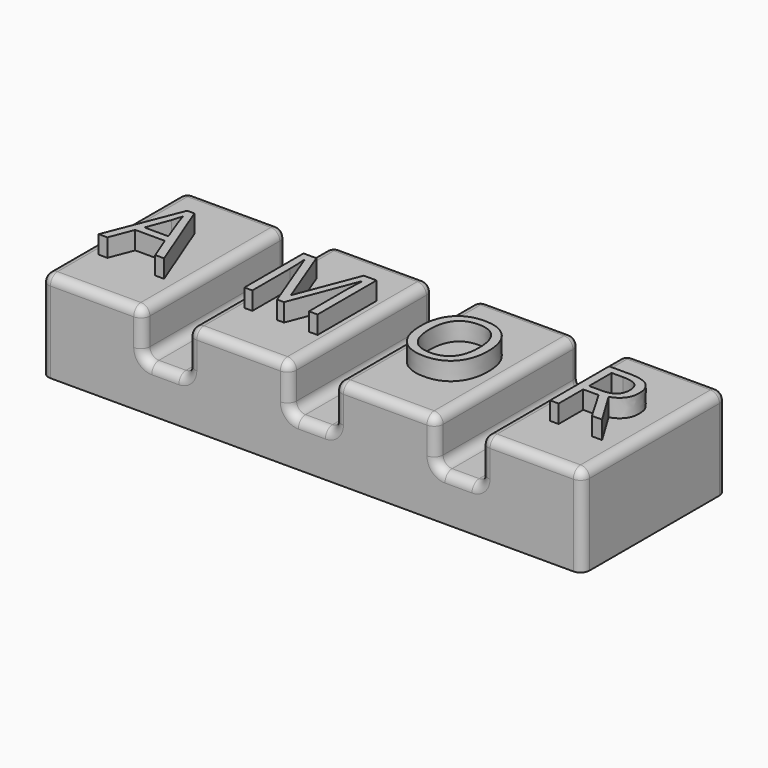
from build123d import *

# Parameters (mm, degrees)
F0_W         = 76.2
F0_H         = 25.4
F1_DEPTH     = 12.7
F2_W         = 6.35
F2_H         = 12.7393246353
F2_H_2       = 12.7
F3_DEPTH     = 25.401
F4_R         = 1.27
F5_T         = -2.54
F6_TEXT_SIZE = 14.5630459127
F10_DEPTH    = 2.54
F7_TEXT_SIZE = 14.5630547222
F11_DEPTH    = 2.54
F8_TEXT_SIZE = 14.5630547222
F12_DEPTH    = 2.54
F9_TEXT_SIZE = 14.5630547222
F13_DEPTH    = 2.54


# Not quite as in the source:
# - Text() gives the source's letters only with a copy of the font that has no kerning and outlines rounded to 1/6400 em; it was checked with that copy


with BuildPart() as f1:
    # F0 (on Top) → F1 (new body)
    with BuildSketch(Plane.XY):
        Rectangle(F0_W, F0_H)
    extrude(amount=F1_DEPTH)

    # F2 (on face) → F3 (cut, through all)
    with BuildSketch(Plane.XZ.offset(12.7)):
        with Locations((0, 12.7)):
            Rectangle(F2_W, F2_H)
        with Locations((-20.6502, 12.7)):
            Rectangle(F2_W, F2_H_2)
        with Locations((20.6502, 12.7)):
            Rectangle(F2_W, F2_H_2)
    extrude(amount=-F3_DEPTH, mode=Mode.SUBTRACT)

    # F4
    f4_edges = [f1.edges().sort_by_distance(p)[0] for p in [
        (-23.8252, 0, 12.7),
        (-30.9626, -12.7, 12.7),
        (-38.1, 0, 12.7),
        (-30.9626, 12.7, 12.7),
        (-3.175, 0, 12.7),
        (-10.3251, -12.7, 12.7),
        (-17.4752, 0, 12.7),
        (-10.3251, 12.7, 12.7),
        (17.4752, 0, 12.7),
        (10.3251, -12.7, 12.7),
        (3.175, 0, 12.7),
        (10.3251, 12.7, 12.7),
        (38.1, 0, 12.7),
        (30.9626, -12.7, 12.7),
        (23.8252, 0, 12.7),
        (30.9626, 12.7, 12.7),
        (-20.6502, -12.7, 6.35),
        (-17.4752, 0, 6.35),
        (-20.6502, 12.7, 6.35),
        (-23.8252, 0, 6.35),
        (0, -12.7, 6.330338),
        (3.175, 0, 6.330338),
        (0, 12.7, 6.330338),
        (-3.175, 0, 6.330338),
        (20.6502, -12.7, 6.35),
        (23.8252, 0, 6.35),
        (20.6502, 12.7, 6.35),
        (17.4752, 0, 6.35),
        (38.1, -12.7, 6.35),
        (38.1, 12.7, 6.35),
        (-38.1, -12.7, 6.35),
        (-38.1, 12.7, 6.35),
        (-23.8252, 12.7, 9.525),
        (-17.4752, 12.7, 9.525),
        (-3.175, 12.7, 9.515169),
        (3.175, 12.7, 9.515169),
        (17.4752, 12.7, 9.525),
        (23.8252, 12.7, 9.525),
        (-23.8252, -12.7, 9.525),
        (-17.4752, -12.7, 9.525),
        (-3.175, -12.7, 9.515169),
        (3.175, -12.7, 9.515169),
        (17.4752, -12.7, 9.525),
        (23.8252, -12.7, 9.525),
    ]]
    fillet(f4_edges, radius=F4_R)

    # F5
    f5_openings = [f1.faces().sort_by_distance(p)[0] for p in [
        (0, 0, 0),
    ]]
    offset(amount=F5_T, openings=f5_openings)

    # F6 (on face) → F10 (join)
    with BuildSketch(Plane.XY.offset(12.7)):
        with Locations((-35.8322989196, -5.4455220853)):
            Text('A', F6_TEXT_SIZE, font='Open Sans', text_align=(TextAlign.LEFT, TextAlign.BOTTOM))
    extrude(amount=F10_DEPTH)

    # F7 (on face) → F11 (join)
    with BuildSketch(Plane.XY.offset(12.7)):
        with Locations((-16.8114297403, -5.3460751583)):
            Text('M', F7_TEXT_SIZE, font='Open Sans', text_align=(TextAlign.LEFT, TextAlign.BOTTOM))
    extrude(amount=F11_DEPTH)

    # F8 (on face) → F12 (join)
    with BuildSketch(Plane.XY.offset(12.7)):
        with Locations((4.5674320779, -5.6118774115)):
            Text('O', F8_TEXT_SIZE, font='Open Sans', text_align=(TextAlign.LEFT, TextAlign.BOTTOM))
    extrude(amount=F12_DEPTH)

    # F9 (on face) → F13 (join)
    with BuildSketch(Plane.XY.offset(12.7)):
        with Locations((26.2375993772, -5.3460172446)):
            Text('R', F9_TEXT_SIZE, font='Open Sans', text_align=(TextAlign.LEFT, TextAlign.BOTTOM))
    extrude(amount=F13_DEPTH)


solid = f1.part
